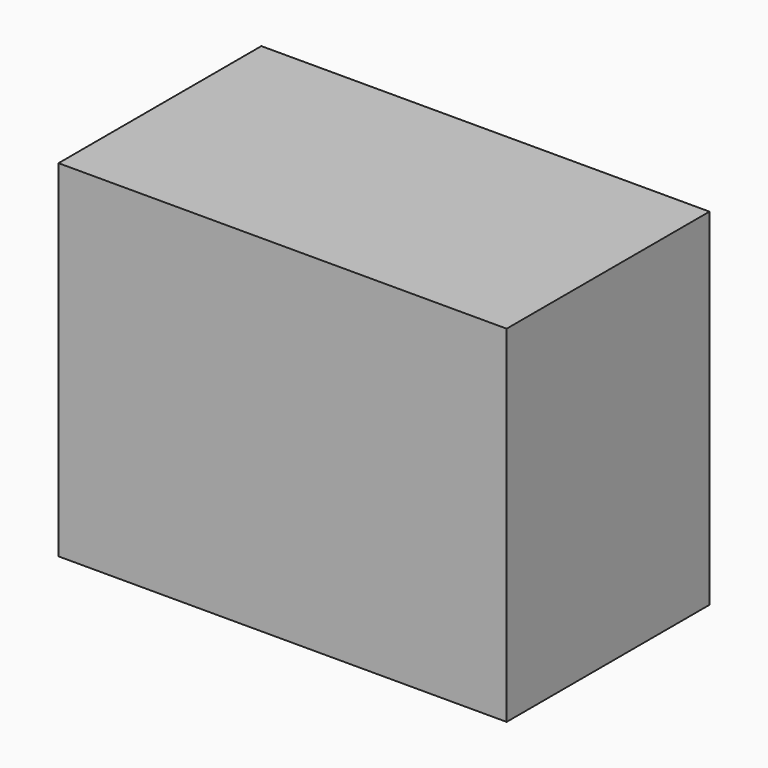
from build123d import *

# Parameters (mm, degrees)
F0_W     = 44.894259423
F0_H     = 34.683033824
F1_DEPTH = 25.4


# Not quite as in the source:
# - the program builds the solid bodies; features that only make, move or delete a surface that nothing else refers to are left out


with BuildPart() as f1:
    # F0 (on Front) → F1 (new body)
    with BuildSketch(Plane.XZ):
        with Locations((22.4471297115, -17.341516912)):
            Rectangle(F0_W, F0_H)
    extrude(amount=F1_DEPTH)


solid = f1.part
